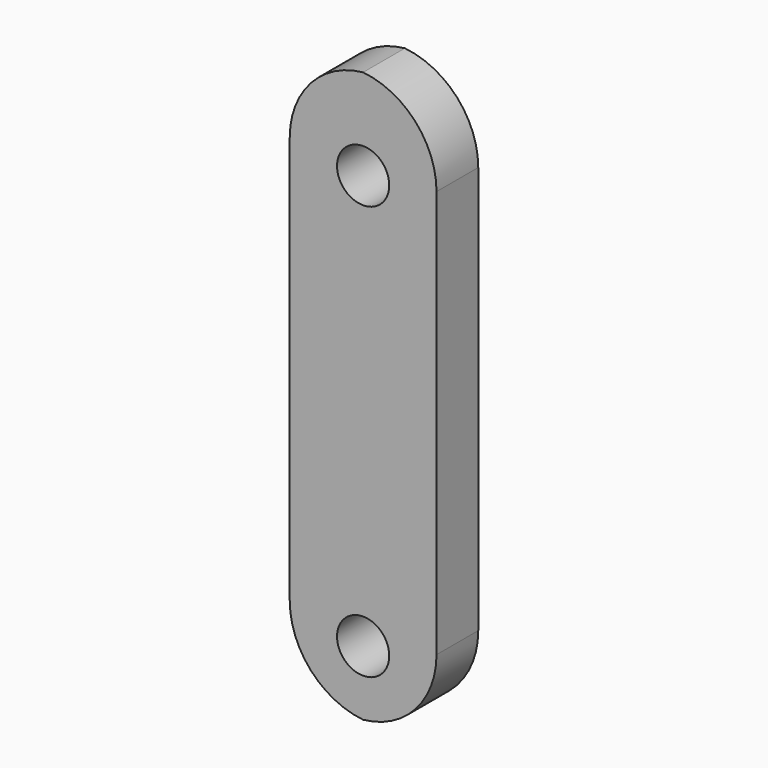
from build123d import *

# Parameters (mm, degrees)
F0_W        = 9
F0_H        = 35
F0_R        = 1.6
F1_DEPTH    = 3.2
F2_T1_DEPTH = 28.2


# Not quite as in the source:
# - a fillet or chamfer that OpenCascade refuses, or shapes differently, is made with other operations: its cross-section is extruded or revolved along the edge and cut away or added


with BuildPart() as f1:
    # F0 (on Front) → F1 (new body)
    with BuildSketch(Plane.XZ):
        with Locations((-14.7368423641, 13.5)):
            Rectangle(F0_W, F0_H)
        with Locations((-14.7368423641, 0)):
            Circle(F0_R, mode=Mode.SUBTRACT)
        with Locations((-14.7368423641, 25.4)):
            Circle(F0_R, mode=Mode.SUBTRACT)
    extrude(amount=F1_DEPTH)

    # F2: fillet of radius 5 on 4 edges, made by hand

    # F2_s2 → F2_t1 (cut)
    with BuildSketch(Plane.XZ.offset(-12.5)):
        with BuildLine():
            ThreePointArc((-10.2368423641, 26), (-11.7013084581, 29.5355339059), (-15.2368423641, 31))
            Line((-15.2368423641, 31), (-10.2368423641, 31))
            Line((-10.2368423641, 31), (-10.2368423641, 26))
        make_face()
        with BuildLine():
            ThreePointArc((-14.2368423641, 31), (-17.77237627, 29.5355339059), (-19.2368423641, 26))
            Line((-19.2368423641, 26), (-19.2368423641, 31))
            Line((-19.2368423641, 31), (-14.2368423641, 31))
        make_face()
        with BuildLine():
            ThreePointArc((-10.2368423641, 1), (-11.7013084581, -2.5355339059), (-15.2368423641, -4))
            Line((-15.2368423641, -4), (-10.2368423641, -4))
            Line((-10.2368423641, -4), (-10.2368423641, 1))
        make_face()
        with BuildLine():
            ThreePointArc((-19.2368423641, 1), (-17.77237627, -2.5355339059), (-14.2368423641, -4))
            Line((-14.2368423641, -4), (-19.2368423641, -4))
            Line((-19.2368423641, -4), (-19.2368423641, 1))
        make_face()
    extrude(amount=F2_T1_DEPTH, mode=Mode.SUBTRACT)


solid = f1.part
